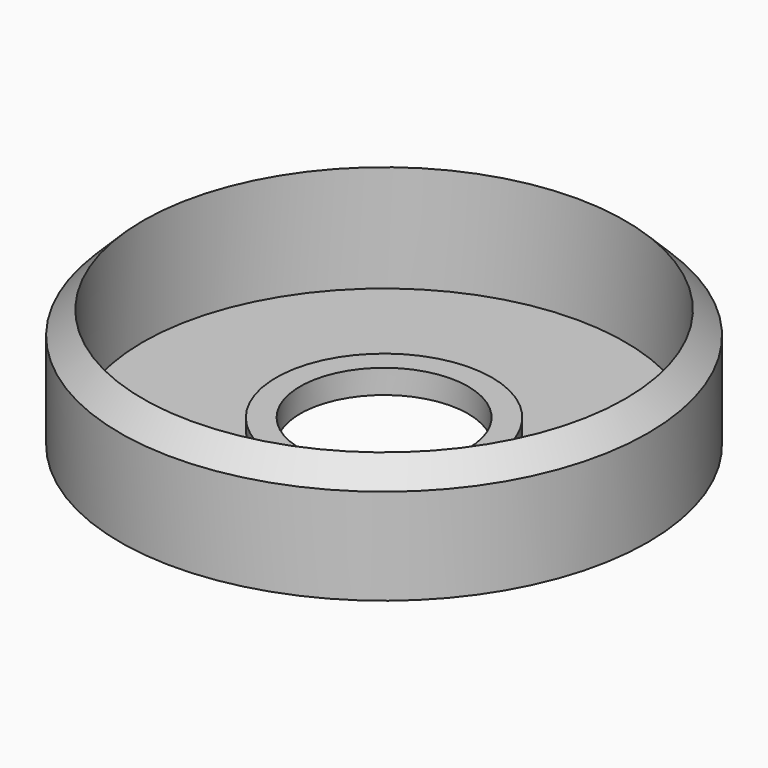
from build123d import *

# Parameters (mm, degrees)
F0_R     = 11
F0_R_2   = 10.5
F0_R_3   = 10.05
F1_DEPTH = 5
F0_R_4   = 4.5
F6_DEPTH = 0.5
F0_R_5   = 3.5
F7_DEPTH = 1


# Not quite as in the source:
# - a fillet or chamfer that OpenCascade refuses, or shapes differently, is made with other operations: its cross-section is extruded or revolved along the edge and cut away or added


with BuildPart() as f1:
    # F0 (on Top) → F1 (new body)
    with BuildSketch(Plane.XY):
        Circle(F0_R)
        Circle(F0_R_2, mode=Mode.SUBTRACT)
        Circle(F0_R_2)
        Circle(F0_R_3, mode=Mode.SUBTRACT)
    extrude(amount=F1_DEPTH)

    # F5: chamfer of 1 on 1 edges, made by hand

    # F5_s1 → F5_t2 (revolve, cut)
    with BuildSketch(Plane.XZ):
        Polygon((11, 4), (10, 5), (11, 5), align=None)
    revolve(axis=Axis((0, 0, 5), (0, 0, 1)), mode=Mode.SUBTRACT)

    # F0 (on Top) → F6 (join)
    with BuildSketch(Plane.XY):
        Circle(F0_R_3)
        Circle(F0_R_4, mode=Mode.SUBTRACT)
    extrude(amount=F6_DEPTH)

    # F0 (on Top) → F7 (join)
    with BuildSketch(Plane.XY):
        Circle(F0_R_4)
        Circle(F0_R_5, mode=Mode.SUBTRACT)
    extrude(amount=F7_DEPTH)


solid = f1.part
